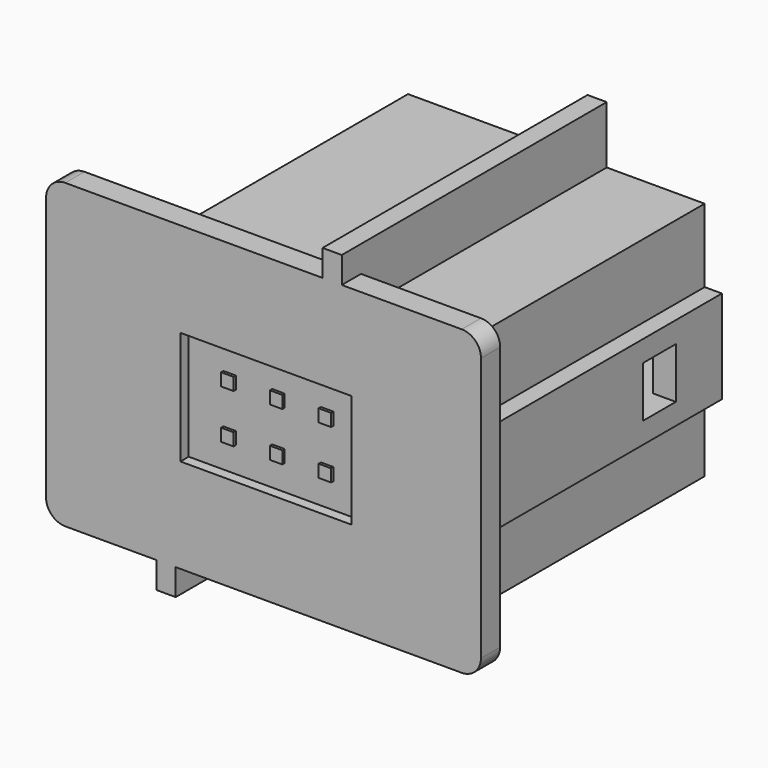
from build123d import *

# Parameters (mm, degrees)
F0_W          = 1
F0_H          = 1.375
F1_DEPTH      = 16
F0_W_2        = 0.65
F0_H_2        = 0.65
F2_DEPTH      = 1.25
F3_W          = 2.15
F3_H          = 2.65
F4_DEPTH      = 1.2
F5_R          = 1
F6_W          = 8.9
F6_H          = 5.9
F7_DEPTH      = 0.5
F7_TAPER      = 3
F8_DEPTH      = 7
F8_DEPTH_BACK = 0.9
F9_SIZE       = 0.3


# Not quite as in the source:
# - a feature names something its author has since deleted; it is built from what else it names


with BuildPart() as f1:
    # F0 (on Front) → F1 (new body)
    with BuildSketch(Plane.XZ):
        Polygon((-1.15, 11.35), (-1.15, -1.15), (-0.45, -1.15), (-0.45, -2.775), (0.55, -2.775), (0.55, -1.15), (14.3, -1.15), (14.3, 2.675), (15.2, 2.675), (15.2, 7.525), (14.3, 7.525), (14.3, 11.35), (9.2, 11.35), (9.2, 12.975), (8.2, 12.975), (8.2, 11.35), align=None)
        Polygon((13.2, 0), (0, 0), (0, 10), (11, 10), (11, 8.325), (13.2, 8.325), (13.2, 7.425), (11, 7.425), (11, 6.425), (14, 6.425), (14, 3.775), (11, 3.775), (11, 0.9), (13.2, 0.9), align=None, mode=Mode.SUBTRACT)
        with Locations((8.7, 13.6625)):
            Rectangle(F0_W, F0_H)
        with Locations((0.05, -3.4625)):
            Rectangle(F0_W, F0_H)
    extrude(amount=-F1_DEPTH)

    # F0 (on Front) → F2 (join)
    with BuildSketch(Plane.XZ):
        Polygon((-1.15, 11.35), (-1.15, -1.15), (-0.45, -1.15), (-0.45, -2.775), (0.55, -2.775), (0.55, -1.15), (14.3, -1.15), (14.3, 2.675), (15.2, 2.675), (15.2, 7.525), (14.3, 7.525), (14.3, 11.35), (9.2, 11.35), (9.2, 12.975), (8.2, 12.975), (8.2, 11.35), align=None)
        Polygon((13.2, 0), (0, 0), (0, 10), (11, 10), (11, 8.325), (13.2, 8.325), (13.2, 7.425), (11, 7.425), (11, 6.425), (14, 6.425), (14, 3.775), (11, 3.775), (11, 0.9), (13.2, 0.9), align=None, mode=Mode.SUBTRACT)
        Polygon((-0.45, -1.15), (-1.15, -1.15), (-1.15, 11.35), (8.2, 11.35), (8.2, 12.975), (-6.2, 12.975), (-6.2, -2.775), (-0.45, -2.775), align=None)
        with Locations((0.05, -3.4625)):
            Rectangle(F0_W, F0_H)
        Polygon((0.55, -1.15), (0.55, -2.775), (16.45, -2.775), (16.45, 12.975), (9.2, 12.975), (9.2, 11.35), (14.3, 11.35), (14.3, 7.525), (15.2, 7.525), (15.2, 2.675), (14.3, 2.675), (14.3, -1.15), align=None)
        with Locations((8.7, 13.6625)):
            Rectangle(F0_W, F0_H)
        Polygon((0, 10), (0, 0), (13.2, 0), (13.2, 0.9), (11, 0.9), (11, 3.775), (14, 3.775), (14, 6.425), (11, 6.425), (11, 7.425), (13.2, 7.425), (13.2, 8.325), (11, 8.325), (11, 10), align=None)
        with Locations((2.96, 3.83)):
            Rectangle(F0_W_2, F0_H_2, mode=Mode.SUBTRACT)
        with Locations((5.5, 3.83)):
            Rectangle(F0_W_2, F0_H_2, mode=Mode.SUBTRACT)
        with Locations((8.04, 3.83)):
            Rectangle(F0_W_2, F0_H_2, mode=Mode.SUBTRACT)
        with Locations((2.96, 6.37)):
            Rectangle(F0_W_2, F0_H_2, mode=Mode.SUBTRACT)
        with Locations((5.5, 6.37)):
            Rectangle(F0_W_2, F0_H_2, mode=Mode.SUBTRACT)
        with Locations((8.04, 6.37)):
            Rectangle(F0_W_2, F0_H_2, mode=Mode.SUBTRACT)
    extrude(amount=F2_DEPTH)

    # F3 (on face) → F4 (cut, through all)
    with BuildSketch(Plane.YZ.offset(15.2)):
        with Locations((11.925, 5.1)):
            Rectangle(F3_W, F3_H)
    extrude(amount=-F4_DEPTH, mode=Mode.SUBTRACT)

    # F5
    f5_edges = [f1.edges().sort_by_distance(p)[0] for p in [
        (16.45, -0.625, 12.975),
        (-6.2, -0.625, 12.975),
        (16.45, -0.625, -2.775),
        (-6.2, -0.625, -2.775),
    ]]
    fillet(f5_edges, radius=F5_R)

    # F6 (on face) → F7 (cut)
    with BuildSketch(Plane.XZ.offset(1.25)):
        with Locations((5.25, 5.1)):
            Rectangle(F6_W, F6_H)
    extrude(amount=-F7_DEPTH, taper=F7_TAPER, mode=Mode.SUBTRACT)

    # F0 (on Front) → F8 (join, two sides)
    with BuildSketch(Plane.XZ) as f8_sk:
        with Locations((2.96, 6.37)):
            Rectangle(F0_W_2, F0_H_2)
        with Locations((5.5, 6.37)):
            Rectangle(F0_W_2, F0_H_2)
        with Locations((8.04, 6.37)):
            Rectangle(F0_W_2, F0_H_2)
        with Locations((2.96, 3.83)):
            Rectangle(F0_W_2, F0_H_2)
        with Locations((5.5, 3.83)):
            Rectangle(F0_W_2, F0_H_2)
        with Locations((8.04, 3.83)):
            Rectangle(F0_W_2, F0_H_2)
    extrude(amount=-F8_DEPTH)
    extrude(f8_sk.sketch, amount=F8_DEPTH_BACK)

    # F9
    f9_edges = [f1.edges().sort_by_distance(p)[0] for p in [
        (12.1, 16, 7.425),
        (13.2, 16, 7.875),
        (5.5, 16, 10),
        (0, 16, 5),
        (6.6, 16, 0),
        (12.1, 16, 0.9),
        (13.2, 16, 0.45),
        (11, 16, 2.3375),
        (12.5, 16, 3.775),
        (14, 16, 5.1),
        (12.5, 16, 6.425),
        (11, 16, 6.925),
        (12.1, 16, 8.325),
        (11, 16, 9.1625),
    ]]
    chamfer(f9_edges, length=F9_SIZE)


solid = f1.part
